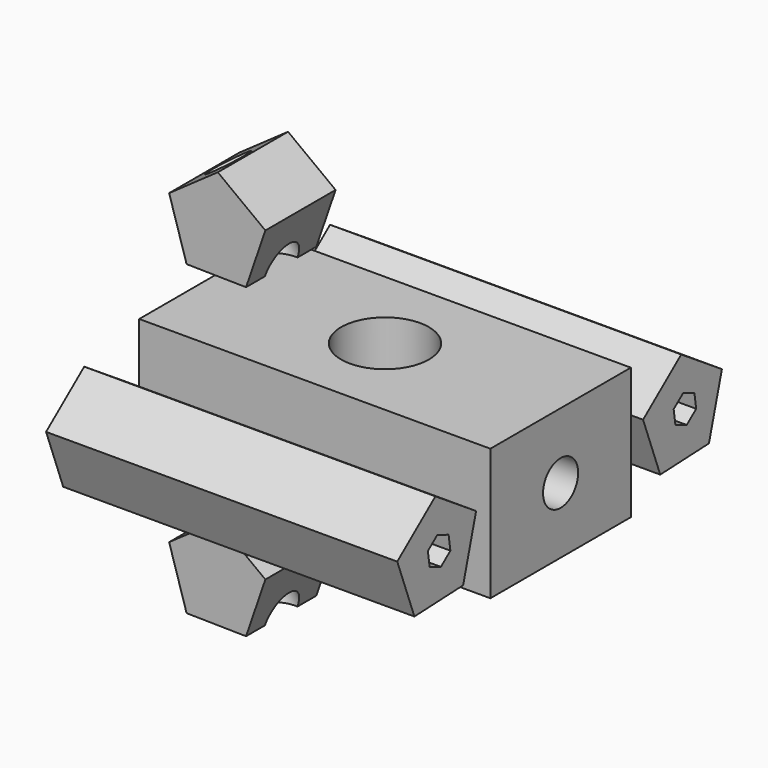
from build123d import *

# Parameters (mm, degrees)
F0_W      = 101.6
F0_H      = 50.8
F1_DEPTH  = 19.05
F2_R      = 12.7
F3_DEPTH  = 38.101
F4_R      = 6.35
F5_DEPTH  = 50.8
F7_DEPTH  = 12.7
F10_R     = 5.9048963233
F11_DEPTH = 112.0212777668
F13_DEPTH = 50.8
F15_DEPTH = 103.0949723509


# Not quite as in the source:
# - the program builds the solid bodies; features that only make, move or delete a surface that nothing else refers to are left out


with BuildPart() as f1:
    # F0 (on Top) → F1 (new body, symmetric)
    with BuildSketch(Plane.XY):
        Rectangle(F0_W, F0_H)
    extrude(amount=F1_DEPTH, both=True)

    # F2 (on face) → F3 (cut, through all)
    with BuildSketch(Plane.XY.offset(19.05)):
        Circle(F2_R)
    extrude(amount=-F3_DEPTH, mode=Mode.SUBTRACT)

    # F4 (on face) → F5 (cut)
    with BuildSketch(Plane.YZ.offset(50.8)):
        Circle(F4_R)
    extrude(amount=-F5_DEPTH, mode=Mode.SUBTRACT)


with BuildPart() as f7:
    # F6 (on Front) → F7 (new body, symmetric)
    with BuildSketch(Plane.XZ):
        Polygon((-47.2491934158, 29.014438658), (-30.0442731298, 28.7286156648), (-24.4558265543, 45.0031430529), (-38.2068969123, 55.3471771228), (-52.2939723509, 45.4656143707), align=None)
    extrude(amount=F7_DEPTH, both=True)

    # F10 (on face) → F11 (cut, through all)
    with BuildSketch(Plane(origin=(-38.6204902945, 0, 55.0570566519), x_dir=(0.8186688273, 0, 0.5742659238), z_dir=(-0.5742659238, 0, 0.8186688273))):
        with Locations((-8.2643283531, 0)):
            Circle(F10_R)
    extrude(amount=-F11_DEPTH, mode=Mode.SUBTRACT)


with BuildPart() as f13:
    # F12 (on Right) → F13 (new body, symmetric)
    with BuildSketch(Plane.YZ):
        Polygon((53.6531691035, -11.7309192025), (58.3421756071, 5.2770554258), (43.6156132043, 14.9923188161), (29.8250905982, 3.9887071727), (36.0286413079, -12.5271622122), align=None)
    extrude(amount=F13_DEPTH, both=True)

    # F14 (on face) → F15 (cut, through all)
    with BuildSketch(Plane.YZ.offset(50.8)):
        Polygon((40.8914412669, 2.1650664507), (41.5386756608, -2.1650664507), (45.6122979522, -3.7696114741), (49.0386858496, -1.0440235961), (48.3914514557, 3.2861093053), (44.3178291644, 4.8906543287), align=None)
    extrude(amount=-F15_DEPTH, mode=Mode.SUBTRACT)


with BuildPart() as f16_1:
    # F16: copy of F13
    add(f13.part.moved(Location((0, -88.9, 0))))


with BuildPart() as f17_1:
    # F17: copy of F7
    add(f7.part.moved(Location((0, 0, -88.9))))


solid = Compound([f1.part, f7.part, f13.part, f16_1.part, f17_1.part])
